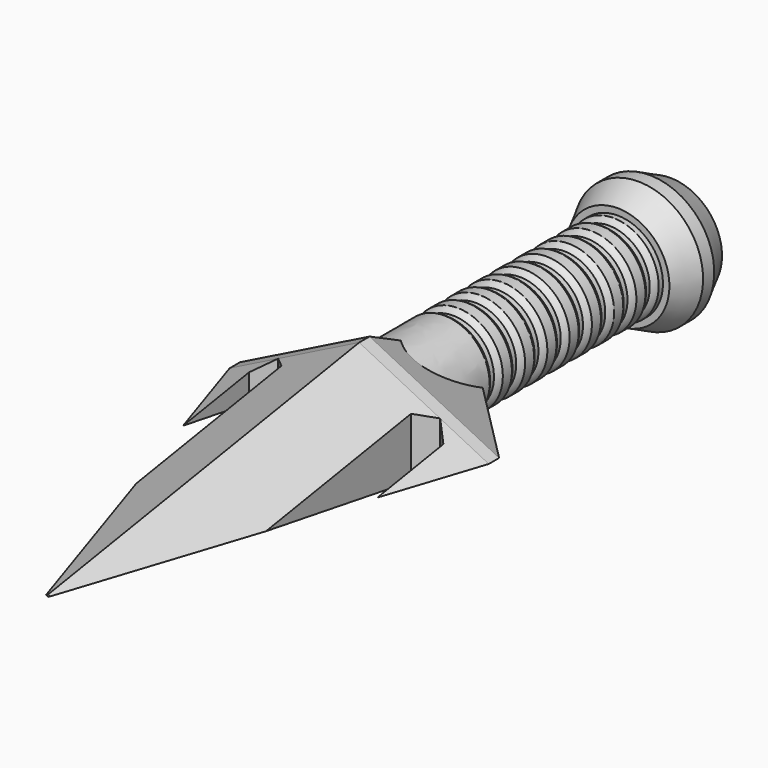
from build123d import *

# Parameters (mm, degrees)
F11_DEPTH      = 76.2
F0_SIZE2       = 11.17599
F0_SIZE        = 76.19999
F1_DEPTH       = 25.4
F2_SIZE2       = 22.86
F2_SIZE        = 10.16
F3_DEPTH       = 76.2
F4_SIZE        = 2.54
F5_W           = 6.35
F5_H           = 61.6873274763
F13_DEPTH      = 25.4
F13_DEPTH_BACK = 25.4
F14_SIZE       = 3.17499
F7_R           = 12.7
F8_DEPTH       = 12.8905
F9_SIZE2       = 2.54
F9_SIZE        = 5.08


# Not quite as in the source:
# - a fillet or chamfer is up to 0.001 mm smaller than in the source, because OpenCascade refuses the exact size


with BuildPart() as f11:
    # F10 (on Front) → F11 (new body)
    with BuildSketch(Plane.XZ):
        Polygon((25.4, 0), (0, 12.7), (-25.4, 0), (0, -12.7), align=None)
    extrude(amount=F11_DEPTH)

    # F0 (size 76.2 and 11.176 in the source; OpenCascade refuses exactly that, so slightly less here)
    f0_edges = [f11.edges().sort_by_distance(p)[0] for p in [
        (12.7, -76.2, 6.35),
        (-12.7, -76.2, 6.35),
        (-12.7, -76.2, -6.35),
        (12.7, -76.2, -6.35),
    ]]
    chamfer(f0_edges, length=F0_SIZE, length2=F0_SIZE2)

    # F1 (add): a face of the model
    f1_faces = [f11.faces().sort_by_distance(p)[0] for p in [
        (0, 0, 0),
    ]]
    extrude(f1_faces, amount=F1_DEPTH)

    # F2
    f2_edges = [f11.edges().sort_by_distance(p)[0] for p in [
        (12.7, 25.4, 6.35),
        (-12.7, 25.4, 6.35),
        (-12.7, 25.4, -6.35),
        (12.7, 25.4, -6.35),
    ]]
    f2_side = f11.faces().sort_by_distance((0, 25.4, 0))[0]
    chamfer(f2_edges, length=F2_SIZE, length2=F2_SIZE2, reference=f2_side)

    # F12 (on Front) → F3 (join)
    with BuildSketch(Plane.XZ):
        with BuildLine():
            add(Edge.make_bspline(
                [(-8.89, 0), (-8.89, -15.3979316793), (4.445, -7.6989658396), (17.78, 0), (4.445, 7.6989658396), (-8.89, 15.3979316793), (-8.89, 0)],
                knots=[0, 0, 0, 2.0943951024, 2.0943951024, 4.1887902048, 4.1887902048, 6.2831853072, 6.2831853072, 6.2831853072], degree=2, weights=[1, 0.5, 1, 0.5, 1, 0.5, 1]))
        make_face()
    extrude(amount=-F3_DEPTH)

    # F4
    f4_edges = [f11.edges().sort_by_distance(p)[0] for p in [
        (8.89, 76.2, 0),
    ]]
    chamfer(f4_edges, length=F4_SIZE)

    # F5 (on Top) → F13 (cut, two sides)
    with BuildSketch(Plane.XY) as f13_sk:
        with Locations((-15.875, -30.8436637381)):
            Rectangle(F5_W, F5_H)
        with Locations((15.875, -30.8436637381)):
            Rectangle(F5_W, F5_H)
    extrude(amount=-F13_DEPTH, mode=Mode.SUBTRACT)
    extrude(f13_sk.sketch, amount=F13_DEPTH_BACK, mode=Mode.SUBTRACT)

    # F14 (size 3.175 in the source; OpenCascade refuses exactly that, so slightly less here)
    f14_edges = [f11.edges().sort_by_distance(p)[0] for p in [
        (12.7, 0, 0),
        (19.05, 0, 0),
        (-12.7, 0, 0),
        (-19.05, 0, 0),
    ]]
    chamfer(f14_edges, length=F14_SIZE)

    # F16 (on Top) → F6 (revolve, cut)
    with BuildSketch(Plane.XY):
        with BuildLine():
            Line((-9.125418961, 62.2203871608), (-9.125418961, 57.9181527479))
            ThreePointArc((-9.125418961, 57.9181527479), (-8.8331419916, 59.1465062454), (-8.018955113, 60.1115854486))
            Line((-8.018955113, 60.1115854486), (-8.018955113, 61.1794027921))
            ThreePointArc((-8.018955113, 61.1794027921), (-8.8331419916, 62.1444819954), (-9.125418961, 63.3728354929))
            Line((-9.125418961, 63.3728354929), (-9.125418961, 62.2203871608))
        make_face()
        with BuildLine():
            Line((-9.125418961, 57.9181527479), (-9.125418961, 52.4634698497))
            ThreePointArc((-9.125418961, 52.4634698497), (-8.8331419916, 53.6918233472), (-8.018955113, 54.6569025504))
            Line((-8.018955113, 54.6569025504), (-8.018955113, 55.7247200471))
            ThreePointArc((-8.018955113, 55.7247200471), (-8.8331419916, 56.6897992503), (-9.125418961, 57.9181527479))
        make_face()
        with BuildLine():
            Line((-9.125418961, 52.4634698497), (-9.125418961, 47.008787256))
            ThreePointArc((-9.125418961, 47.008787256), (-8.8331419916, 48.2371407535), (-8.018955113, 49.2022199567))
            Line((-8.018955113, 49.2022199567), (-8.018955113, 50.2700371489))
            ThreePointArc((-8.018955113, 50.2700371489), (-8.8331419916, 51.2351163521), (-9.125418961, 52.4634698497))
        make_face()
        with BuildLine():
            Line((-9.125418961, 47.008787256), (-9.125418961, 41.5541043587))
            ThreePointArc((-9.125418961, 41.5541043587), (-8.8331419916, 42.7824578562), (-8.018955113, 43.7475370594))
            Line((-8.018955113, 43.7475370594), (-8.018955113, 44.8153545552))
            ThreePointArc((-8.018955113, 44.8153545552), (-8.8331419916, 45.7804337584), (-9.125418961, 47.008787256))
        make_face()
        with BuildLine():
            Line((-9.125418961, 41.5541043587), (-9.125418961, 36.0994217608))
            ThreePointArc((-9.125418961, 36.0994217608), (-8.8331419924, 37.3277752601), (-8.018955113, 38.2928544648))
            Line((-8.018955113, 38.2928544648), (-8.018955113, 39.3606716579))
            ThreePointArc((-8.018955113, 39.3606716579), (-8.8331419916, 40.3257508611), (-9.125418961, 41.5541043587))
        make_face()
        with BuildLine():
            Line((-9.125418961, 36.0994217608), (-9.125418961, 30.644739044))
            ThreePointArc((-9.125418961, 30.644739044), (-8.8331419916, 31.8730925415), (-8.018955113, 32.8381717447))
            Line((-8.018955113, 32.8381717447), (-8.018955113, 33.9059890633))
            ThreePointArc((-8.018955113, 33.9059890633), (-8.8331419909, 34.871068265), (-9.125418961, 36.0994217608))
        make_face()
        with BuildLine():
            Line((-9.125418961, 30.644739044), (-9.125418961, 25.1900562989))
            ThreePointArc((-9.125418961, 25.1900562989), (-8.8331419916, 26.4184097965), (-8.018955113, 27.3834889997))
            Line((-8.018955113, 27.3834889997), (-8.018955113, 28.4513063432))
            ThreePointArc((-8.018955113, 28.4513063432), (-8.8331419916, 29.4163855464), (-9.125418961, 30.644739044))
        make_face()
        with BuildLine():
            Line((-9.125418961, 25.1900562989), (-9.125418961, 19.735373578))
            ThreePointArc((-9.125418961, 19.735373578), (-8.8331419916, 20.9637270756), (-8.018955113, 21.9288062788))
            Line((-8.018955113, 21.9288062788), (-8.018955113, 22.9966235981))
            ThreePointArc((-8.018955113, 22.9966235981), (-8.8331419916, 23.9617028014), (-9.125418961, 25.1900562989))
        make_face()
    revolve(axis=Axis((0, 0.2972502261, 0), (0, 1, 0)), mode=Mode.SUBTRACT)

    # F7 (on face) → F8 (join)
    with BuildSketch(Plane(origin=(0, 76.2, 0), x_dir=(-1, 0, 0), z_dir=(0, 1, 0))):
        Circle(F7_R)
        with BuildLine():
            add(Edge.make_bspline(
                [(6.35, 0), (6.35, -0.9165435523), (6.2055816016, -1.9165462182), (5.8743687497, -2.9685787155), (5.3096370214, -4.0303567141), (4.4903381982, -5.0017671596), (3.4092421438, -5.8432871327), (2.1249952321, -6.3393982068), (0.8786810279, -6.5578157966), (-0.3140856404, -6.5381100219), (-1.3811067413, -6.3302774805), (-2.3224274554, -5.9914943022), (-4.0275725446, -5.0070283259), (-4.7916225874, -4.3612341238), (-5.500221654, -3.5437644787), (-6.1015307125, -2.5291827692), (-6.5236530355, -1.350015893), (-6.7207764555, 0), (-6.5236530355, 1.350015893), (-6.1015307125, 2.5291827692), (-5.500221654, 3.5437644787), (-4.7916225874, 4.3612341238), (-4.0275725446, 5.0070283259), (-2.3224274554, 5.9914943022), (-1.3811067413, 6.3302774805), (-0.3140856404, 6.5381100219), (0.8786810279, 6.5578157966), (2.124995232, 6.3393982068), (3.4092421438, 5.8432871328), (4.4903381982, 5.0017671596), (5.3096370214, 4.0303567141), (5.8743687497, 2.9685787155), (6.2055816016, 1.9165462182), (6.35, 0.9165435523), (6.35, 0)],
                knots=[0, 0, 0, 0, 0, 0, 0, 0, 0, 0, 0, 0, 0, 18.6191724603, 18.6191724603, 18.6191724603, 18.6191724603, 18.6191724603, 18.6191724603, 18.6191724603, 18.6191724603, 18.6191724603, 18.6191724603, 18.6191724603, 37.2383449206, 37.2383449206, 37.2383449206, 37.2383449206, 37.2383449206, 37.2383449206, 37.2383449206, 37.2383449206, 37.2383449206, 37.2383449206, 37.2383449206, 55.8575173808, 55.8575173808, 55.8575173808, 55.8575173808, 55.8575173808, 55.8575173808, 55.8575173808, 55.8575173808, 55.8575173808, 55.8575173808, 55.8575173808, 55.8575173808, 55.8575173808], degree=12))
        make_face(mode=Mode.SUBTRACT)
    extrude(amount=-F8_DEPTH)

    # F9
    f9_edges = [f11.edges().sort_by_distance(p)[0] for p in [
        (12.7, 63.3095, 0),
        (12.7, 76.2, 0),
    ]]
    f9_side = f11.faces().sort_by_distance((12.7, 69.75475, 0))[0]
    chamfer(f9_edges, length=F9_SIZE, length2=F9_SIZE2, reference=f9_side)


solid = f11.part
